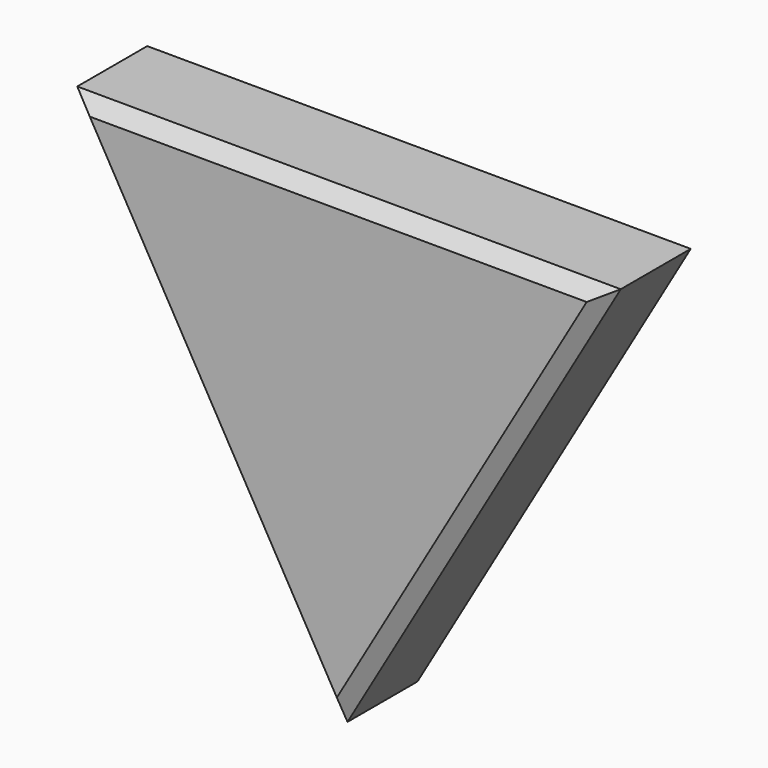
from build123d import *

# Parameters (mm, degrees)
F1_DEPTH = 15
F2_SIZE  = 2
F3_SCALE = 0.5


with BuildPart() as f1:
    # F0 (on Front) → F1 (new body)
    with BuildSketch(Plane.XZ):
        Polygon((-0.1495843466, -46.6474431687), (40.472662979, 23.1941777401), (-40.3230786324, 23.4532654285), align=None)
    extrude(amount=F1_DEPTH)

    # F2
    f2_edges = [f1.edges().sort_by_distance(p)[0] for p in [
        (0.074792, -15, 23.323722),
        (20.161539, -15, -11.726633),
        (-20.236331, -15, -11.597089),
    ]]
    chamfer(f2_edges, length=F2_SIZE)


with BuildPart() as f1_1:
    # F3: moved
    add(f1.part.scale(F3_SCALE))


solid = f1_1.part
